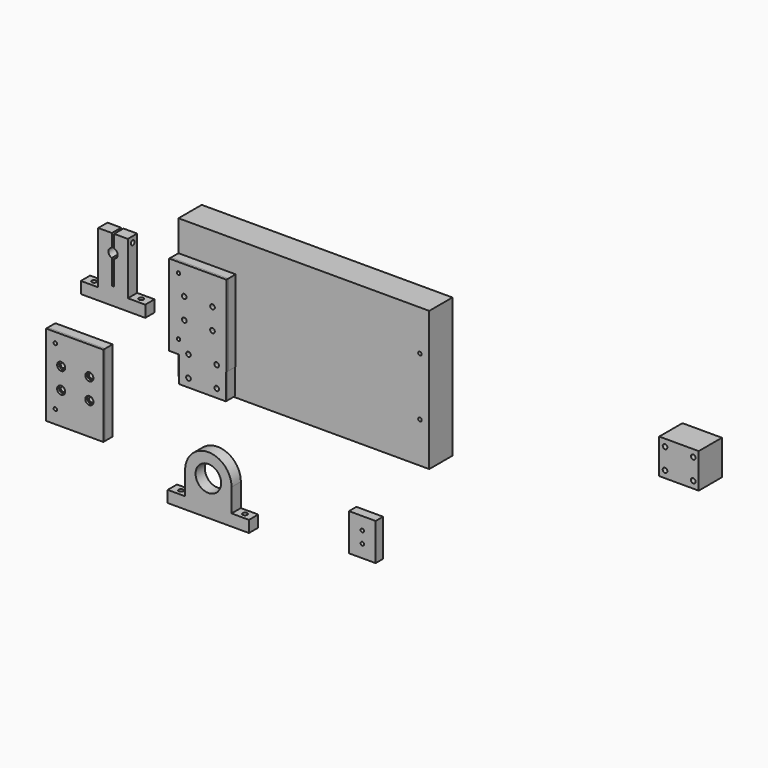
from build123d import *
from build123d import SkipClean  # not in build123d's __all__

# Parameters (mm, degrees)
F0_R      = 11
F1_DEPTH  = 10
F2_R      = 2
F3_DEPTH  = 25
F4_DEPTH  = 10
F5_R      = 2
F6_DEPTH  = 36.2
F8_R      = 2
F7_R      = 2
F9_DEPTH  = 25
F10_W     = 10
F10_H     = 30
F10_R     = 2
F10_W_2   = 14
F11_DEPTH = 25
F10_W_3   = 216
F10_H_2   = 120
F10_R_2   = 1.5
F12_R     = 2
F12_R_2   = 1.5
F12_W     = 40.2169972658
F12_H     = 22.4555346966
F13_DEPTH = 10
F12_W_2   = 49.3000489473
F12_H_2   = 70
F14_R     = 3.5
F15_DEPTH = 5
F0_W      = 23
F0_H      = 32
F0_R_2    = 1.5
F16_DEPTH = 8


# Not quite as in the source:
# - a feature names something its author has since deleted; it is built from what else it names


with BuildPart() as f1:
    # F0 (on Front) → F1 (new body)
    with BuildSketch(Plane.XZ):
        with BuildLine():
            ThreePointArc((-210.1082575321, -138.1097745895), (-230.1082575321, -118.1097745895), (-250.1082575321, -138.1097745895))
            Line((-250.1082575321, -138.1097745895), (-250.1082575321, -158.1097745895))
            Line((-250.1082575321, -158.1097745895), (-265.1082575321, -158.1097745895))
            Line((-265.1082575321, -158.1097745895), (-265.1082575321, -168.1097745895))
            Line((-265.1082575321, -168.1097745895), (-195.1082575321, -168.1097745895))
            Line((-195.1082575321, -168.1097745895), (-195.1082575321, -158.1097745895))
            Line((-195.1082575321, -158.1097745895), (-210.1082575321, -158.1097745895))
            Line((-210.1082575321, -158.1097745895), (-210.1082575321, -138.1097745895))
        make_face()
        with Locations((-230.1082575321, -138.1097745895)):
            Circle(F0_R, mode=Mode.SUBTRACT)
    extrude(amount=F1_DEPTH)

    # F2 (on face) → F3 (cut)
    with BuildSketch(Plane.XY.offset(-158.1097745895)):
        with Locations((-257.6082575321, -5)):
            Circle(F2_R)
        with Locations((-202.6082575321, -5)):
            Circle(F2_R)
    extrude(amount=-F3_DEPTH, mode=Mode.SUBTRACT)


with BuildPart() as f4:
    # F0 (on Front) → F4 (new body)
    with BuildSketch(Plane.XZ):
        with BuildLine():
            Line((-313.1871948242, 21.0148020371), (-324.9384198033, 21.0148020371))
            Line((-324.9384198033, 21.0148020371), (-324.9384198033, -23.9851979629))
            Line((-324.9384198033, -23.9851979629), (-339.9384198033, -23.9851979629))
            Line((-339.9384198033, -23.9851979629), (-339.9384198033, -33.9851979629))
            Line((-339.9384198033, -33.9851979629), (-284.4359698451, -33.9851979629))
            Line((-284.4359698451, -33.9851979629), (-284.4359698451, -23.9851979629))
            Line((-284.4359698451, -23.9851979629), (-299.4359698451, -23.9851979629))
            Line((-299.4359698451, -23.9851979629), (-299.4359698451, 21.0148020371))
            Line((-299.4359698451, 21.0148020371), (-311.1871948242, 21.0148020371))
            Line((-311.1871948242, 21.0148020371), (-311.1871948242, 9.8877853833))
            ThreePointArc((-311.1871948242, 9.8877853833), (-309.0249171641, 8.4642917799), (-308.1871948242, 6.0148020371))
            ThreePointArc((-308.1871948242, 6.0148020371), (-309.0249171641, 3.5653122943), (-311.1871948242, 2.1418186909))
            Line((-311.1871948242, 2.1418186909), (-311.1871948242, -18.9851979629))
            Line((-311.1871948242, -18.9851979629), (-313.1871948242, -18.9851979629))
            Line((-313.1871948242, -18.9851979629), (-313.1871948242, 2.1418186909))
            ThreePointArc((-313.1871948242, 2.1418186909), (-316.1871948242, 6.0148020371), (-313.1871948242, 9.8877853833))
            Line((-313.1871948242, 9.8877853833), (-313.1871948242, 21.0148020371))
        make_face()
    extrude(amount=F4_DEPTH)

    # F5 (on face) → F6 (cut)
    with BuildSketch(Plane(origin=(-324.9384198033, 0, 0), x_dir=(0, -1, 0), z_dir=(-1, 0, 0))):
        with Locations((4.7623808496, 16.0148020371)):
            Circle(F5_R)
    extrude(amount=-F6_DEPTH, mode=Mode.SUBTRACT)

    # F8 (on face) + F7 (on face) → F9 (cut)
    with BuildSketch(Plane.XY.offset(-23.9851979629)):
        with Locations((-291.9359698451, -5)):
            Circle(F8_R)
    with BuildSketch(Plane.XY.offset(-23.9851979629)):
        with Locations((-332.4384198033, -5)):
            Circle(F7_R)
    extrude(amount=-F9_DEPTH, mode=Mode.SUBTRACT)


with BuildPart() as f11:
    # F10 (on Front) → F11 (new body)
    with BuildSketch(Plane.XZ):
        with Locations((175.29543221, 15)):
            Rectangle(F10_W, F10_H)
        with Locations((175.29543221, 6)):
            Circle(F10_R, mode=Mode.SUBTRACT)
        with Locations((175.29543221, 24)):
            Circle(F10_R, mode=Mode.SUBTRACT)
        with Locations((199.29543221, 15)):
            Rectangle(F10_W, F10_H)
        with Locations((199.5954811573, 6)):
            Circle(F10_R, mode=Mode.SUBTRACT)
        with Locations((199.5954811573, 24)):
            Circle(F10_R, mode=Mode.SUBTRACT)
        with Locations((187.29543221, 15)):
            Rectangle(F10_W_2, F10_H)
    extrude(amount=F11_DEPTH)


with BuildPart() as f11b:
    # F10 (on Front) → F11, piece 2 (new body)
    with BuildSketch(Plane.XZ):
        with Locations((-135.8186649084, 0.8761131763)):
            Rectangle(F10_W_3, F10_H_2)
        with Locations((-235.8186649084, -24.1238868237)):
            Circle(F10_R_2, mode=Mode.SUBTRACT)
        Polygon((-235.8186649084, -14.1238868237), (-235.8186649084, 15.8761131763), (-225.8186649084, 15.8761131763), (-211.8186649084, 15.8761131763), (-201.8186649084, 15.8761131763), (-201.8186649084, -14.1238868237), (-211.8186649084, -14.1238868237), (-225.8186649084, -14.1238868237), align=None, mode=Mode.SUBTRACT)
        with Locations((-35.8186649084, -24.1238868237)):
            Circle(F10_R_2, mode=Mode.SUBTRACT)
        with Locations((-235.8186649084, 25.8761131763)):
            Circle(F10_R_2, mode=Mode.SUBTRACT)
        with Locations((-35.8186649084, 25.8761131763)):
            Circle(F10_R_2, mode=Mode.SUBTRACT)
        with Locations((-230.8186649084, 0.8761131763)):
            Rectangle(F10_W, F10_H)
        with Locations((-230.8186649084, -8.1238868237)):
            Circle(F10_R, mode=Mode.SUBTRACT)
        with Locations((-230.8186649084, 9.8761131763)):
            Circle(F10_R, mode=Mode.SUBTRACT)
        with Locations((-218.8186649084, 0.8761131763)):
            Rectangle(F10_W_2, F10_H)
        with Locations((-206.8186649084, 0.8761131763)):
            Rectangle(F10_W, F10_H)
        with Locations((-206.5186159611, -8.1238868237)):
            Circle(F10_R, mode=Mode.SUBTRACT)
        with Locations((-206.5186159611, 9.8761131763)):
            Circle(F10_R, mode=Mode.SUBTRACT)
    extrude(amount=F11_DEPTH)

    # F12 (on face) → F13 (join)
    with BuildSketch(Plane.XZ.offset(25)):
        with BuildLine():
            Line((-194.5186159611, -35.6238868237), (-194.5186159611, 34.3761131763))
            Line((-194.5186159611, 34.3761131763), (-243.8186649084, 34.3761131763))
            Line((-243.8186649084, 34.3761131763), (-243.8186649084, -35.6238868237))
            Line((-243.8186649084, -35.6238868237), (-235.2415621281, -35.6238868237))
            Line((-235.2415621281, -35.6238868237), (-235.2415621281, -25.5084273182))
            ThreePointArc((-235.2415621281, -25.5084273182), (-237.0667943429, -23.2919175245), (-234.3186649084, -24.1238868237))
            ThreePointArc((-234.3186649084, -24.1238868237), (-234.4434145104, -24.7227911088), (-234.7969133655, -25.2220779657))
            Line((-234.7969133655, -25.2220779657), (-195.0245648623, -25.2220779657))
            Line((-195.0245648623, -25.2220779657), (-195.0245648623, -35.6238868237))
            Line((-195.0245648623, -35.6238868237), (-194.5186159611, -35.6238868237))
        make_face()
        with Locations((-230.8186649084, -8.1238868237)):
            Circle(F12_R, mode=Mode.SUBTRACT)
        with Locations((-206.5186159611, -8.1238868237)):
            Circle(F12_R, mode=Mode.SUBTRACT)
        with Locations((-235.8186649084, 25.8761131763)):
            Circle(F12_R_2, mode=Mode.SUBTRACT)
        with Locations((-230.8186649084, 9.8761131763)):
            Circle(F12_R, mode=Mode.SUBTRACT)
        with Locations((-206.5186159611, 9.8761131763)):
            Circle(F12_R, mode=Mode.SUBTRACT)
        with Locations((-215.1330634952, -46.8516541719)):
            Rectangle(F12_W, F12_H)
        with Locations((-227.2052568197, -50.8580457568)):
            Circle(F12_R, mode=Mode.SUBTRACT)
        with Locations((-202.9052078724, -50.8580457568)):
            Circle(F12_R, mode=Mode.SUBTRACT)
        with BuildLine():
            Line((-235.2415621281, -35.6238868237), (-195.0245648623, -35.6238868237))
            Line((-195.0245648623, -35.6238868237), (-195.0245648623, -25.2220779657))
            Line((-195.0245648623, -25.2220779657), (-234.7969133655, -25.2220779657))
            ThreePointArc((-234.7969133655, -25.2220779657), (-235.006517893, -25.3850042747), (-235.2415621281, -25.5084273182))
            Line((-235.2415621281, -25.5084273182), (-235.2415621281, -35.6238868237))
        make_face()
        with Locations((-227.2052568197, -32.8580457568)):
            Circle(F12_R, mode=Mode.SUBTRACT)
        with Locations((-202.9052078724, -32.8580457568)):
            Circle(F12_R, mode=Mode.SUBTRACT)
    with SkipClean():  # cleaning this boolean's faces spoils the solid; the shape is the same uncleaned
        extrude(amount=F13_DEPTH)


with BuildPart() as f13:
    # F12 (on face) → F13, piece 2 (new body)
    with BuildSketch(Plane.XZ.offset(25)):
        with Locations((-325.2200314403, -88.2029348612)):
            Rectangle(F12_W_2, F12_H_2)
        with Locations((-341.8700559139, -111.7029348612)):
            Circle(F12_R_2, mode=Mode.SUBTRACT)
        with Locations((-336.8700559139, -95.7029348612)):
            Circle(F12_R, mode=Mode.SUBTRACT)
        with Locations((-312.5700069666, -95.7029348612)):
            Circle(F12_R, mode=Mode.SUBTRACT)
        with Locations((-336.8700559139, -77.7029348612)):
            Circle(F12_R, mode=Mode.SUBTRACT)
        with Locations((-312.5700069666, -77.7029348612)):
            Circle(F12_R, mode=Mode.SUBTRACT)
        with Locations((-341.8700559139, -61.7029348612)):
            Circle(F12_R_2, mode=Mode.SUBTRACT)
    extrude(amount=F13_DEPTH)

    # F14 (on face) → F15 (cut)
    with BuildSketch(Plane.XZ.offset(35)):
        with Locations((-336.8700559139, -77.7029348612)):
            Circle(F14_R)
        with Locations((-312.5700069666, -77.7029348612)):
            Circle(F14_R)
        with Locations((-336.8700559139, -95.7029348612)):
            Circle(F14_R)
        with Locations((-312.5700069666, -95.7029348612)):
            Circle(F14_R)
    extrude(amount=-F15_DEPTH, mode=Mode.SUBTRACT)


with BuildPart() as f16:
    # F0 (on Front) → F16 (new body)
    with BuildSketch(Plane.XZ):
        with Locations((-99.0838845968, -140.7919552326)):
            Rectangle(F0_W, F0_H)
        with Locations((-99.0838845968, -145.7919552326)):
            Circle(F0_R_2, mode=Mode.SUBTRACT)
        with Locations((-99.0838845968, -135.7919552326)):
            Circle(F0_R_2, mode=Mode.SUBTRACT)
    extrude(amount=F16_DEPTH)


with BuildPart() as f16b:
    # F12 (on face) → F16, piece 2 (new body)
    with BuildSketch(Plane.XZ.offset(25)):
        with BuildLine():
            Line((-194.5186159611, -35.6238868237), (-194.5186159611, 34.3761131763))
            Line((-194.5186159611, 34.3761131763), (-243.8186649084, 34.3761131763))
            Line((-243.8186649084, 34.3761131763), (-243.8186649084, -35.6238868237))
            Line((-243.8186649084, -35.6238868237), (-235.2415621281, -35.6238868237))
            Line((-235.2415621281, -35.6238868237), (-235.2415621281, -25.5084273182))
            ThreePointArc((-235.2415621281, -25.5084273182), (-237.0667943429, -23.2919175245), (-234.3186649084, -24.1238868237))
            ThreePointArc((-234.3186649084, -24.1238868237), (-234.4434145104, -24.7227911088), (-234.7969133655, -25.2220779657))
            Line((-234.7969133655, -25.2220779657), (-195.0245648623, -25.2220779657))
            Line((-195.0245648623, -25.2220779657), (-195.0245648623, -35.6238868237))
            Line((-195.0245648623, -35.6238868237), (-194.5186159611, -35.6238868237))
        make_face()
        with Locations((-230.8186649084, -8.1238868237)):
            Circle(F12_R, mode=Mode.SUBTRACT)
        with Locations((-206.5186159611, -8.1238868237)):
            Circle(F12_R, mode=Mode.SUBTRACT)
        with Locations((-235.8186649084, 25.8761131763)):
            Circle(F12_R_2, mode=Mode.SUBTRACT)
        with Locations((-230.8186649084, 9.8761131763)):
            Circle(F12_R, mode=Mode.SUBTRACT)
        with Locations((-206.5186159611, 9.8761131763)):
            Circle(F12_R, mode=Mode.SUBTRACT)
        with Locations((-215.1330634952, -46.8516541719)):
            Rectangle(F12_W, F12_H)
        with Locations((-227.2052568197, -50.8580457568)):
            Circle(F12_R, mode=Mode.SUBTRACT)
        with Locations((-202.9052078724, -50.8580457568)):
            Circle(F12_R, mode=Mode.SUBTRACT)
        with BuildLine():
            Line((-235.2415621281, -35.6238868237), (-195.0245648623, -35.6238868237))
            Line((-195.0245648623, -35.6238868237), (-195.0245648623, -25.2220779657))
            Line((-195.0245648623, -25.2220779657), (-234.7969133655, -25.2220779657))
            ThreePointArc((-234.7969133655, -25.2220779657), (-235.006517893, -25.3850042747), (-235.2415621281, -25.5084273182))
            Line((-235.2415621281, -25.5084273182), (-235.2415621281, -35.6238868237))
        make_face()
        with Locations((-227.2052568197, -32.8580457568)):
            Circle(F12_R, mode=Mode.SUBTRACT)
        with Locations((-202.9052078724, -32.8580457568)):
            Circle(F12_R, mode=Mode.SUBTRACT)
    extrude(amount=F16_DEPTH)


with BuildPart() as f16c:
    # F12 (on face) → F16, piece 3 (new body)
    with BuildSketch(Plane.XZ.offset(25)):
        with Locations((-325.2200314403, -88.2029348612)):
            Rectangle(F12_W_2, F12_H_2)
        with Locations((-341.8700559139, -111.7029348612)):
            Circle(F12_R_2, mode=Mode.SUBTRACT)
        with Locations((-336.8700559139, -95.7029348612)):
            Circle(F12_R, mode=Mode.SUBTRACT)
        with Locations((-312.5700069666, -95.7029348612)):
            Circle(F12_R, mode=Mode.SUBTRACT)
        with Locations((-336.8700559139, -77.7029348612)):
            Circle(F12_R, mode=Mode.SUBTRACT)
        with Locations((-312.5700069666, -77.7029348612)):
            Circle(F12_R, mode=Mode.SUBTRACT)
        with Locations((-341.8700559139, -61.7029348612)):
            Circle(F12_R_2, mode=Mode.SUBTRACT)
    extrude(amount=F16_DEPTH)


solid = Compound([f1.part, f4.part, f11.part, f11b.part, f13.part, f16.part, f16b.part, f16c.part])
